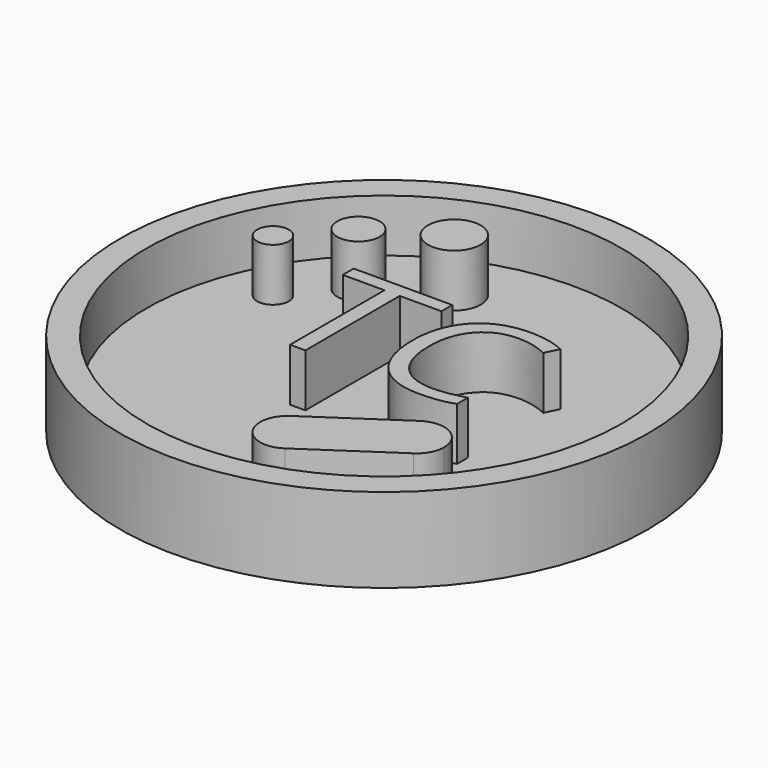
from build123d import *

# Parameters (mm, degrees)
F0_R         = 25
F0_R_2       = 22.5
F0_R_3       = 1.5
F0_R_4       = 2
F0_R_5       = 2.5
F0_TEXT_SIZE = 17.4601141933
F1_DEPTH     = 5
F2_R         = 25
F3_DEPTH     = 3


# Not quite as in the source:
# - Text() gives the source's letters only with a copy of the font that has no kerning and outlines rounded to 1/6400 em; it was checked with that copy


with BuildPart() as f1:
    # F0 (on Top) → F1 (new body)
    with BuildSketch(Plane.XY):
        Circle(F0_R)
        Circle(F0_R_2, mode=Mode.SUBTRACT)
        with Locations((-16.4741910994, 7.4392203242)):
            Circle(F0_R_3)
        with Locations((-12.1815605089, 12.1917780489)):
            Circle(F0_R_4)
        with Locations((-6.0492269695, 15.8711783588)):
            Circle(F0_R_5)
        with BuildLine():
            ThreePointArc((13.4521596114, -13.3098967026), (9.8334065388, -12.5992038052), (10.5440994362, -8.9804507326))
            Line((10.5440994362, -8.9804507326), (2.6050617896, -14.3130497232))
            ThreePointArc((2.6050617896, -14.3130497232), (5.2855743778, -14.1764752974), (6.6668167664, -16.4777727082))
            ThreePointArc((6.6668167664, -16.4777727082), (6.3603892881, -17.7042552088), (5.5131219649, -18.6424956932))
            Line((5.5131219649, -18.6424956932), (13.4521596114, -13.3098967026))
        make_face()
        with BuildLine():
            ThreePointArc((6.6668167664, -16.4777727082), (5.2855743778, -14.1764752974), (2.6050617896, -14.3130497232))
            ThreePointArc((2.6050617896, -14.3130497232), (1.8943688923, -17.9318027959), (5.5131219649, -18.6424956932))
            ThreePointArc((5.5131219649, -18.6424956932), (6.3603892881, -17.7042552088), (6.6668167664, -16.4777727082))
        make_face()
        with BuildLine():
            ThreePointArc((13.4521596114, -13.3098967026), (14.2994269347, -12.3716562181), (14.6058544129, -11.1451737176))
            ThreePointArc((14.6058544129, -11.1451737176), (13.2246120244, -8.8438763067), (10.5440994362, -8.9804507326))
            ThreePointArc((10.5440994362, -8.9804507326), (9.8334065388, -12.5992038052), (13.4521596114, -13.3098967026))
        make_face()
        with Locations((-8.6554693989, -5.4386785778)):
            Text('TC', F0_TEXT_SIZE, font='Open Sans', text_align=(TextAlign.LEFT, TextAlign.BOTTOM))
    extrude(amount=F1_DEPTH)

    # F2 (on Top) → F3 (join)
    with BuildSketch(Plane.XY):
        Circle(F2_R)
    extrude(amount=-F3_DEPTH)


solid = f1.part
